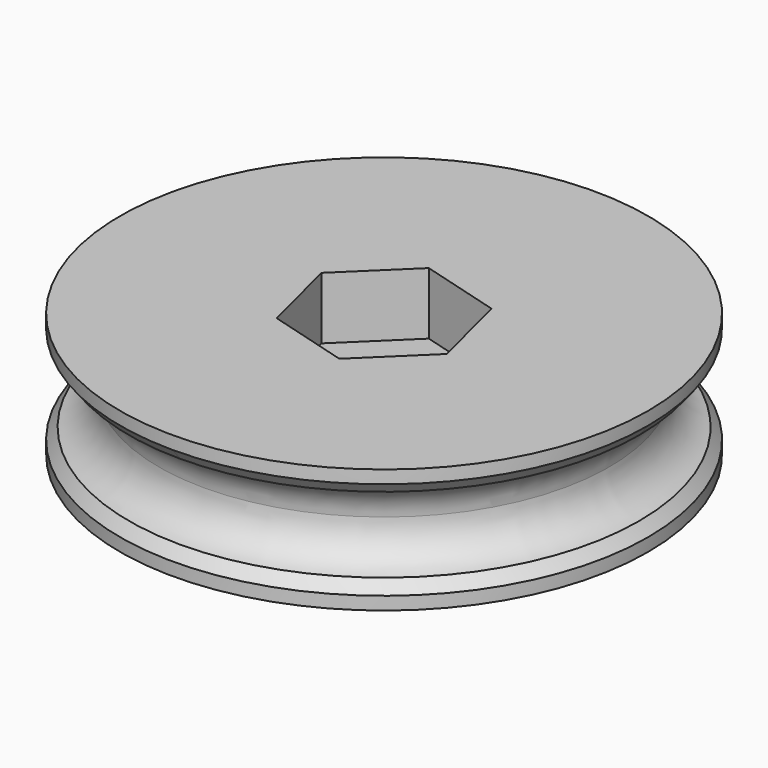
from build123d import *

# Parameters (mm, degrees)
F0_R        = 17
F1_DEPTH    = 4
F2_R        = 2.5
F3_DEPTH    = 25
F5_DEPTH    = 4
F6_R        = 2.5
F8_T2_ANGLE = 270
F8_T4_ANGLE = 90
F8_T6_ANGLE = 90
F8_T8_ANGLE = 270


# Not quite as in the source:
# - a fillet or chamfer that OpenCascade refuses, or shapes differently, is made with other operations: its cross-section is extruded or revolved along the edge and cut away or added


with BuildPart() as f1:
    # F0 (on Top) → F1 (new body, symmetric)
    with BuildSketch(Plane.XY):
        Circle(F0_R)
    extrude(amount=F1_DEPTH, both=True)

    # F2 (on face) → F3 (cut)
    with BuildSketch(Plane.XY.offset(4)):
        Circle(F2_R)
    extrude(amount=-F3_DEPTH, mode=Mode.SUBTRACT)

    # F4 (on face) → F5 (cut)
    with BuildSketch(Plane.XY.offset(4)):
        Polygon((5.2209928438, -1.4814071211), (3.8934326221, 3.7808088751), (-1.3275602216, 5.2622159963), (-5.2209928438, 1.4814071211), (-3.8934326221, -3.7808088751), (1.3275602216, -5.2622159963), align=None)
    extrude(amount=-F5_DEPTH, mode=Mode.SUBTRACT)

    # F6 (on Right) → F7 (revolve, cut)
    with BuildSketch(Plane.YZ):
        with Locations((-17, 0)):
            Circle(F6_R)
    revolve(axis=Axis((0, 0, 0), (0, 0, 1)), mode=Mode.SUBTRACT)

    # F8: chamfer of 0.75 on 4 edges, made by hand

    # F8_s1 → F8_t2 (revolve, cut)
    with BuildSketch(Plane.YZ):
        with BuildLine():
            Line((-17, -3.1622776602), (-16.4230769231, -2.4325212771))
            ThreePointArc((-16.4230769231, -2.4325212771), (-16.6989227011, -2.4818042751), (-17, -2.5))
            Line((-17, -2.5), (-17, -3.1622776602))
        make_face()
    revolve(axis=Axis((0, 0, -2.5), (0, 0, -1)), revolution_arc=F8_T2_ANGLE, mode=Mode.SUBTRACT)

    # F8_s3 → F8_t4 (revolve, cut)
    with BuildSketch(Plane.XZ):
        with BuildLine():
            Line((17, -3.1622776602), (16.4230769231, -2.4325212771))
            ThreePointArc((16.4230769231, -2.4325212771), (16.6989227011, -2.4818042751), (17, -2.5))
            Line((17, -2.5), (17, -3.1622776602))
        make_face()
    revolve(axis=Axis((0, 0, -2.5), (0, 0, -1)), revolution_arc=F8_T4_ANGLE, mode=Mode.SUBTRACT)

    # F8_s5 → F8_t6 (revolve, cut)
    with BuildSketch(Plane.XZ):
        with BuildLine():
            Line((16.4230769231, 2.4325212771), (17, 3.1622776602))
            Line((17, 3.1622776602), (17, 2.5))
            ThreePointArc((17, 2.5), (16.6989227011, 2.4818042751), (16.4230769231, 2.4325212771))
        make_face()
    revolve(axis=Axis((0, 0, 2.5), (0, 0, -1)), revolution_arc=F8_T6_ANGLE, mode=Mode.SUBTRACT)

    # F8_s7 → F8_t8 (revolve, cut)
    with BuildSketch(Plane.YZ):
        with BuildLine():
            Line((-16.4230769231, 2.4325212771), (-17, 3.1622776602))
            Line((-17, 3.1622776602), (-17, 2.5))
            ThreePointArc((-17, 2.5), (-16.6989227011, 2.4818042751), (-16.4230769231, 2.4325212771))
        make_face()
    revolve(axis=Axis((0, 0, 2.5), (0, 0, -1)), revolution_arc=F8_T8_ANGLE, mode=Mode.SUBTRACT)


solid = f1.part
